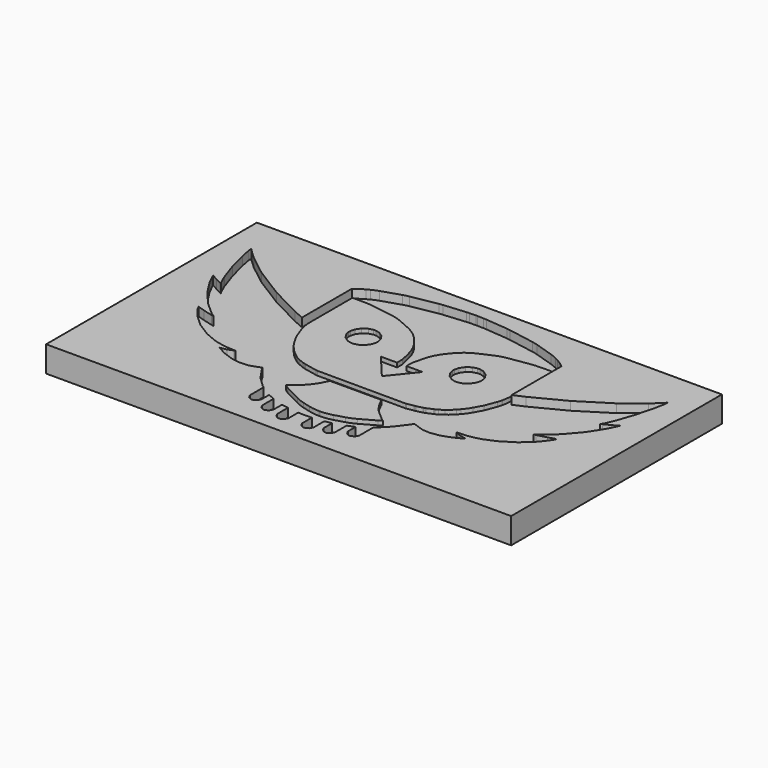
from build123d import *

# Parameters (mm, degrees)
F0_W         = 54.0378913283
F0_H         = 30.6113883853
F1_DEPTH     = 3
F3_DEPTH     = 1
F4_DEPTH     = 0.5
F5_T1_DEPTH  = 1.4279951692
F5_T3_DEPTH  = 1.2750830795
F5_T5_DEPTH  = 1.4154747072
F5_T7_DEPTH  = 1.5538784875
F5_T9_DEPTH  = 1.5346197721
F5_T11_DEPTH = 1.8207083396
F5_T13_DEPTH = 1.842360331
F5_T15_DEPTH = 2.0618682494
F5_T17_DEPTH = 2.9056600537
F5_T19_DEPTH = 2.0631169342
F5_T21_DEPTH = 2.918698365
F5_T23_DEPTH = 2.247874979
F5_T25_DEPTH = 2.5072646643
F5_T27_DEPTH = 3.2701181572
F5_T29_DEPTH = 3.5518654723
F5_T31_DEPTH = 2.1420463635
F5_T33_DEPTH = 3.251600212
F5_T35_DEPTH = 3.5501799152
F5_T37_DEPTH = 2.1451171913
F5_T39_DEPTH = 1.2435255605
F5_T41_DEPTH = 1.2450054051
F5_T43_DEPTH = 2.1117868823
F5_T45_DEPTH = 2.2921133442
F5_T47_DEPTH = 1.9025172431
F5_T49_DEPTH = 1.8626989409
F5_T51_DEPTH = 1.7955373145
F5_T53_DEPTH = 1.8853577819
F5_T55_DEPTH = 1.8365367416
F5_T57_DEPTH = 1.9053253307


# Not quite as in the source:
# - a fillet or chamfer that OpenCascade refuses, or shapes differently, is made with other operations: its cross-section is extruded or revolved along the edge and cut away or added


with BuildPart() as f1:
    # F0 (on Top) → F1 (new body)
    with BuildSketch(Plane.XY):
        Rectangle(F0_W, F0_H)
    extrude(amount=F1_DEPTH)

    # F2 (on face) → F3 (cut)
    with BuildSketch(Plane.XY.offset(3)):
        Polygon((18.8432186, -1.4614652), (18.5729626, -1.5221204), (19.0911226, -1.1666728), (20.5160626, 0.0916432), (21.9755466, 1.7893792), (23.0050086, 3.3946592), (23.5104686, 4.3842432), (23.6539786, 4.7230792), (23.5668566, 4.6707552), (22.9813866, 4.3496992), (22.1975426, 3.9626032), (22.0126306, 3.8757352), (22.2041466, 4.0946832), (22.6712526, 5.1599592), (23.3743246, 7.2338692), (23.9392206, 9.4015052), (24.1762026, 10.6240072), (24.1833146, 10.9671612), (23.9239806, 10.6831892), (22.9346506, 9.7543112), (20.6303626, 7.9450692), (17.1053506, 5.7291732), (13.4495286, 3.8439852), (12.1968006, 3.2940752), (12.1968006, 10.4639872), (12.1968006, 10.5163112), (11.8302786, 10.8884212), (10.3680006, 11.6438172), (7.4962766, 12.5546612), (3.9245286, 13.1899152), (0.9809226, 13.4571232), (-2.54e-05, 13.4807452), (-0.9812274, 13.4611872), (-3.9192708, 13.2008372), (-7.4718418, 12.5655832), (-10.3257604, 11.6466112), (-11.7809518, 10.8871512), (-12.1447814, 10.5163112), (-12.1447814, 10.4901492), (-12.1709688, 10.4901492), (-12.1709688, 3.2940752), (-13.4249668, 3.8439852), (-17.085056, 5.7291732), (-20.618323, 7.9450692), (-22.9320598, 9.7543112), (-23.9256316, 10.6831892), (-24.1833146, 10.9671612), (-24.1778028, 10.6171492), (-23.942167, 9.3905832), (-23.3771694, 7.2229472), (-22.6729798, 5.1558952), (-22.205823, 4.0946832), (-22.014307, 3.8757352), (-22.2003112, 3.9626032), (-22.9706424, 4.3496992), (-23.5425234, 4.6707552), (-23.627969, 4.7230792), (-23.490174, 4.3870372), (-22.9954582, 3.4058352), (-21.9743274, 1.7990312), (-20.517739, 0.0944372), (-19.0942214, -1.1666728), (-18.5747152, -1.5221204), (-18.8461904, -1.4614652), (-19.9472296, -1.1735308), (-20.7175608, -0.9253728), (-20.823682, -0.8867648), (-20.6266288, -1.2754102), (-19.824573, -2.3379176), (-18.458942, -3.5946842), (-16.8618154, -4.588256), (-15.599537, -5.1298094), (-15.1613108, -5.252466), (-14.9297898, -5.3186076), (-13.8783568, -5.5060088), (-12.985369, -5.5487316), (-12.8324102, -5.5432198), (-12.9192274, -5.602478), (-13.5545068, -5.8463942), (-14.214602, -5.9855608), (-14.313789, -5.9924442), (-14.0616432, -6.1509402), (-13.2610098, -6.5629536), (-12.1516648, -6.9653404), (-11.0327186, -7.1376032), (-10.208641, -7.0921372), (-9.948164, -7.0245986), (-9.876536, -7.003923), (-8.917432, -6.6731896), (-8.8113108, -6.6277236), (-8.6404196, -6.9446902), (-7.707503, -8.3048094), (-6.5885314, -9.385173), (-6.3239396, -9.5643192), (-6.3239396, -11.4439954), (-6.3239396, -11.563858), (-6.1323982, -11.9262652), (-5.7809892, -12.1316242), (-5.6624982, -12.1316242), (-5.5453788, -12.1316242), (-5.1939698, -11.9262652), (-5.0010314, -11.563858), (-5.0010314, -11.4439954), (-5.0010314, -10.438003), (-4.9348898, -10.4710738), (-4.273423, -10.7342686), (-4.2072814, -10.7549442), (-4.2072814, -12.3162822), (-4.2072814, -12.4361702), (-4.0157146, -12.7985774), (-3.664331, -13.003911), (-3.5458146, -13.003911), (-3.4286952, -13.003911), (-3.0772862, -12.7985774), (-2.8843732, -12.4361702), (-2.8843732, -12.3162822), (-2.8843732, -11.205591), (-2.8182062, -11.2179608), (-2.1567648, -11.3309654), (-2.0906232, -11.3378742), (-2.0906232, -12.793091), (-2.0906232, -12.9129536), (-1.8990564, -13.2754116), (-1.5476474, -13.4807198), (-1.4291564, -13.4807198), (-1.312037, -13.4807198), (-0.9606534, -13.2754116), (-0.7676134, -12.9129536), (-0.7676134, -12.793091), (-0.7676134, -11.4963448), (-0.7015734, -11.5018566), (-0.2453894, -11.518392), (0.0784606, -11.5225322), (0.2466086, -11.5225322), (0.7535926, -11.5018566), (0.8198866, -11.4963448), (0.8198866, -12.793091), (0.8198866, -12.9129536), (1.0114026, -13.2754116), (1.3626846, -13.4807198), (1.4813026, -13.4807198), (1.5983966, -13.4807198), (1.9496786, -13.2754116), (2.1427186, -12.9129536), (2.1427186, -12.793091), (2.1427186, -11.3378742), (2.2087586, -11.3309654), (2.8704286, -11.2179608), (2.9364686, -11.205591), (2.9364686, -12.3162822), (2.9364686, -12.4361702), (3.1279846, -12.7985774), (3.4795206, -13.003911), (3.5978846, -13.003911), (3.7149786, -13.003911), (4.0665146, -12.7985774), (4.2593006, -12.4361702), (4.2593006, -12.3162822), (4.2593006, -10.7549442), (4.3255946, -10.7287822), (4.9870106, -10.4641904), (5.0530506, -10.438003), (5.0530506, -11.4439954), (5.0530506, -11.563858), (5.2445666, -11.9262652), (5.5961026, -12.1316242), (5.7147206, -12.1316242), (5.8318146, -12.1316242), (6.1830966, -11.9262652), (6.3761366, -11.563858), (6.3761366, -11.4439954), (6.3761366, -9.5643192), (6.5745106, -9.385173), (7.6354686, -8.3048094), (8.6580726, -6.9446902), (8.8371426, -6.6277236), (8.9417906, -6.6731896), (9.8749866, -7.003923), (9.9478846, -7.0245986), (10.2069646, -7.0921372), (11.0309406, -7.1376032), (12.1500646, -6.9653404), (13.2595366, -6.5629536), (14.0598906, -6.1509402), (14.3136366, -5.9924442), (14.2143226, -5.9855608), (13.5516366, -5.8463942), (12.9176526, -5.602478), (12.8323086, -5.5432198), (12.9836926, -5.5487316), (13.8754866, -5.5060088), (14.9280626, -5.3186076), (15.1594566, -5.252466), (15.5953206, -5.1298094), (16.8587166, -4.5923708), (18.4573926, -3.6043108), (19.8213726, -2.3489158), (20.6250286, -1.2782042), (20.8218786, -0.8867648), (20.7157066, -0.9253728), (19.9455786, -1.1735308), align=None)
        Polygon((-5.1278282, -7.5675744), (-5.6363108, -7.2106536), (-5.4778402, -7.1169276), (-4.7598838, -6.5643252), (-4.135628, -5.9194192), (-4.0226488, -5.7816242), (-3.930269, -5.6686196), (-3.5003486, -5.0622708), (-3.0965902, -4.2864532), (-3.0166564, -4.088003), (2.9887926, -4.088003), (3.0672786, -4.2864532), (3.4711386, -5.0622708), (3.9011606, -5.6686196), (3.9948866, -5.7816242), (4.1132506, -5.9263026), (5.4556406, -7.096252), (5.6085486, -7.1830692), (5.2638706, -7.4338942), (3.1142686, -8.6314026), (0.7370826, -9.3273372), (-0.0538734, -9.3273372), (-0.7193534, -9.3273372), (-2.7162252, -8.8036654), align=None, mode=Mode.SUBTRACT)
        Polygon((5.1978306, -3.2542988), (5.1053746, -3.268091), (-5.1333146, -3.2419036), (-5.2986686, -3.221228), (-6.7938396, -2.916682), (-6.933057, -2.871216), (-6.959219, -2.871216), (-6.9798946, -2.871216), (-7.0391274, -2.8450286), (-7.0653402, -2.8450286), (-7.1452486, -2.8174442), (-7.799832, -2.5528524), (-7.8590902, -2.5266904), (-7.8590902, -2.519807), (-7.8797658, -2.500503), (-7.8852776, -2.500503), (-8.2063336, -2.3351236), (-9.0841576, -1.6819626), (-10.0722176, -0.5657088), (-10.8659676, 0.8742172), (-11.360658, 2.2054312), (-11.4833146, 2.6588212), (-11.4971068, 2.7126692), (-11.6156232, 3.0957012), (-11.6156232, 3.2404812), (-11.6156232, 9.9349052), (-10.504932, 9.9349052), (-9.3749114, 9.8922332), (-5.9959748, 9.3588332), (-2.8857448, 7.9780892), (-1.0846308, 5.7235852), (-0.5031994, 3.3258252), (-0.5031994, 2.5264872), (-2.381377, 2.5264872), (0.0784606, -0.4100068), (2.4597106, 2.5264872), (0.5813806, 2.5264872), (0.5854446, 3.3270952), (1.1726926, 5.7235852), (2.9722826, 7.9780892), (6.0769246, 9.3588332), (9.4518226, 9.8922332), (10.5833926, 9.9349052), (11.7200426, 9.9349052), (11.7200426, 3.2404812), (11.7200426, 3.1094172), (11.5739926, 2.7126692), (11.5615466, 2.6588212), (11.4335306, 2.2013672), (10.9275626, 0.8605012), (10.1228906, -0.5850128), (9.1239086, -1.6971264), (8.2336386, -2.3406608), (7.9113126, -2.500503), (7.9042006, -2.5060148), (7.8574646, -2.5266904), (7.7967586, -2.5528524), (7.1630286, -2.8174442), (7.0898766, -2.8450286), (7.0761606, -2.8505404), (6.9699886, -2.8904946), (6.9575426, -2.897378), (6.9313806, -2.897378), (6.8584826, -2.916682), (6.1775086, -3.0958282), (6.1114686, -3.1096204), (6.1046106, -3.1096204), (6.0853066, -3.1096204), (6.0121546, -3.1219902), align=None, mode=Mode.SUBTRACT)
        Polygon((-4.4195238, 4.4297092), (-4.4195238, 4.5909992), (-4.4195238, 4.7507652), (-4.5504354, 5.2262532), (-4.903216, 5.7484772), (-5.4240938, 6.1012832), (-5.9009026, 6.2308232), (-6.0593732, 6.2308232), (-6.2192154, 6.2308232), (-6.6960242, 6.1012832), (-7.216902, 5.7484772), (-7.5696826, 5.2262532), (-7.6992226, 4.7507652), (-7.6992226, 4.5909992), (-7.6992226, 4.4325032), (-7.5696826, 3.9554912), (-7.216902, 3.4332672), (-6.6960242, 3.0804612), (-6.2192154, 2.9496512), (-6.0593732, 2.9496512), (-5.9009026, 2.9496512), (-5.4240938, 3.0763972), (-4.903216, 3.4236152), (-4.5504354, 3.9445692), align=None)
        Polygon((5.8991246, 2.9234892), (6.0591446, 2.9234892), (6.2176406, 2.9234892), (6.6943986, 3.0542992), (7.2153526, 3.4071052), (7.5681586, 3.9280592), (7.6989686, 4.4048172), (7.6989686, 4.5633132), (7.6989686, 4.7230792), (7.5681586, 5.1998372), (7.2153526, 5.7223152), (6.6943986, 6.0751212), (6.2176406, 6.2046612), (6.0591446, 6.2046612), (5.8991246, 6.2046612), (5.4223666, 6.0751212), (4.9001426, 5.7223152), (4.5473366, 5.1998372), (4.4177966, 4.7230792), (4.4177966, 4.5633132), (4.4177966, 4.4048172), (4.5473366, 3.9280592), (4.9001426, 3.4071052), (5.4223666, 3.0542992), align=None)
    extrude(amount=-F3_DEPTH, mode=Mode.SUBTRACT)

    # F4 (cut): faces of the model
    f4_faces = [f1.faces().sort_by_distance(p)[0] for p in [
        (4.6335561224, 8.4234783668, 3),
        (-0.0086091265, -6.6521338784, 3),
    ]]
    extrude(f4_faces, amount=-F4_DEPTH, mode=Mode.SUBTRACT)

    # F5: fillet of radius 5 on 29 edges, made by hand

    # F5_s2 → F5_t1 (join)
    with BuildSketch(Plane.XY.offset(1.5720048308)):
        with BuildLine():
            ThreePointArc((-0.8100633317, 13.4645989611), (-0.9810687986, 13.4582614763), (-1.1517572483, 13.4460759712))
            Line((-1.1517572483, 13.4460759712), (-0.9812274, 13.4611872))
            Line((-0.9812274, 13.4611872), (-0.8100633317, 13.4645989611))
        make_face()
    extrude(amount=F5_T1_DEPTH)

    # F5_s4 → F5_t3 (join)
    with BuildSketch(Plane.XY.offset(1.7249169205)):
        with BuildLine():
            ThreePointArc((0.1099759424, 13.4780962811), (-2.79096e-05, 13.4795346179), (-0.1100367795, 13.4785523767))
            Line((-0.1100367795, 13.4785523767), (-2.54e-05, 13.4807452))
            Line((-2.54e-05, 13.4807452), (0.1099759424, 13.4780962811))
        make_face()
    extrude(amount=F5_T3_DEPTH)

    # F5_s6 → F5_t5 (join)
    with BuildSketch(Plane.XY.offset(1.5845252928)):
        with BuildLine():
            ThreePointArc((1.1464319639, 13.4420989657), (0.9807644678, 13.4543665866), (0.8147808816, 13.4611240234))
            Line((0.8147808816, 13.4611240234), (0.9809226, 13.4571232))
            Line((0.9809226, 13.4571232), (1.1464319639, 13.4420989657))
        make_face()
    extrude(amount=F5_T5_DEPTH)

    # F5_s8 → F5_t7 (join)
    with BuildSketch(Plane.XY.offset(1.4461215125)):
        with BuildLine():
            ThreePointArc((-3.6985841633, 13.2203929921), (-3.918621846, 13.1959742145), (-4.137362893, 13.161839))
            Line((-4.137362893, 13.161839), (-3.9192708, 13.2008372))
            Line((-3.9192708, 13.2008372), (-3.6985841633, 13.2203929921))
        make_face()
    extrude(amount=F5_T7_DEPTH)

    # F5_s10 → F5_t9 (join)
    with BuildSketch(Plane.XY.offset(1.4653802279)):
        with BuildLine():
            ThreePointArc((3.7115563615, 13.2092479116), (3.9239212188, 13.1853847298), (4.1350724232, 13.1524688836))
            Line((4.1350724232, 13.1524688836), (3.9245286, 13.1899152))
            Line((3.9245286, 13.1899152), (3.7115563615, 13.2092479116))
        make_face()
    extrude(amount=F5_T9_DEPTH)

    # F5_s12 → F5_t11 (join)
    with BuildSketch(Plane.XY.offset(1.1792916604)):
        with BuildLine():
            ThreePointArc((7.8091969967, 12.4554101349), (7.4937011449, 12.544208402), (7.1730654496, 12.6121459879))
            Line((7.1730654496, 12.6121459879), (7.4962766, 12.5546612))
            Line((7.4962766, 12.5546612), (7.8091969967, 12.4554101349))
        make_face()
    extrude(amount=F5_T11_DEPTH)

    # F5_s14 → F5_t13 (join)
    with BuildSketch(Plane.XY.offset(1.157639669)):
        with BuildLine():
            ThreePointArc((-7.1401587111, 12.6248932065), (-7.4690995918, 12.5545794677), (-7.7925684671, 12.4623080657))
            Line((-7.7925684671, 12.4623080657), (-7.4718418, 12.5655832))
            Line((-7.4718418, 12.5655832), (-7.1401587111, 12.6248932065))
        make_face()
    extrude(amount=F5_T13_DEPTH)

    # F5_s16 → F5_t15 (join)
    with BuildSketch(Plane.XY.offset(0.9381317506)):
        with BuildLine():
            ThreePointArc((-9.9214566217, 11.7767984631), (-10.3188095179, 11.6299981099), (-10.7023105403, 11.4500908182))
            Line((-10.7023105403, 11.4500908182), (-10.3257604, 11.6466112))
            Line((-10.3257604, 11.6466112), (-9.9214566217, 11.7767984631))
        make_face()
    extrude(amount=F5_T15_DEPTH)

    # F5_s18 → F5_t17 (join)
    with BuildSketch(Plane.XY.offset(0.0943399463)):
        with BuildLine():
            ThreePointArc((-11.1051838212, 11.2398324687), (-11.6479853297, 10.9111234834), (-12.1447814, 10.5163112))
            Line((-12.1447814, 10.5163112), (-11.7809518, 10.8871512))
            Line((-11.7809518, 10.8871512), (-11.1051838212, 11.2398324687))
        make_face()
    extrude(amount=F5_T17_DEPTH)

    # F5_s20 → F5_t19 (join)
    with BuildSketch(Plane.XY.offset(0.9368830658)):
        with BuildLine():
            ThreePointArc((10.7458128931, 11.4486437139), (10.3611047307, 11.627135416), (9.9626544414, 11.7723835652))
            Line((9.9626544414, 11.7723835652), (10.3680006, 11.6438172))
            Line((10.3680006, 11.6438172), (10.7458128931, 11.4486437139))
        make_face()
    extrude(amount=F5_T19_DEPTH)

    # F5_s22 → F5_t21 (join)
    with BuildSketch(Plane.XY.offset(0.081301635)):
        with BuildLine():
            ThreePointArc((12.1968006, 10.5163112), (11.695774938, 10.9120249966), (11.1484083318, 11.2406675397))
            Line((11.1484083318, 11.2406675397), (11.8302786, 10.8884212))
            Line((11.8302786, 10.8884212), (12.1968006, 10.5163112))
        make_face()
    extrude(amount=F5_T21_DEPTH)

    # F5_s24 → F5_t23 (cut)
    with BuildSketch(Plane.XY.offset(2)):
        with BuildLine():
            ThreePointArc((-11.6156232, 3.7948511916), (-11.5859057875, 3.2505250026), (-11.4971068, 2.7126692))
            Line((-11.4971068, 2.7126692), (-11.6156232, 3.0957012))
            Line((-11.6156232, 3.0957012), (-11.6156232, 3.7948511916))
        make_face()
    extrude(amount=F5_T23_DEPTH, mode=Mode.SUBTRACT)

    # F5_s26 → F5_t25 (cut)
    with BuildSketch(Plane.XY.offset(2)):
        with BuildLine():
            ThreePointArc((11.7200426, 3.9123230657), (11.6833958012, 3.3080673251), (11.5739926, 2.7126692))
            Line((11.5739926, 2.7126692), (11.7200426, 3.1094172))
            Line((11.7200426, 3.1094172), (11.7200426, 3.9123230657))
        make_face()
    extrude(amount=F5_T25_DEPTH, mode=Mode.SUBTRACT)

    # F5_s28 → F5_t27 (cut)
    with BuildSketch(Plane.XY.offset(2)):
        with BuildLine():
            ThreePointArc((-0.8235085604, 4.6467454195), (-1.1935422662, 5.670169038), (-1.7762394596, 6.5892908074))
            Line((-1.7762394596, 6.5892908074), (-1.0846308, 5.7235852))
            Line((-1.0846308, 5.7235852), (-0.8235085604, 4.6467454195))
        make_face()
    extrude(amount=F5_T27_DEPTH, mode=Mode.SUBTRACT)

    # F5_s30 → F5_t29 (cut)
    with BuildSketch(Plane.XY.offset(2)):
        with BuildLine():
            ThreePointArc((-2.1237929739, 7.0243331136), (-2.9754726001, 7.8618209534), (-4.0014870822, 8.4734077011))
            Line((-4.0014870822, 8.4734077011), (-2.8857448, 7.9780892))
            Line((-2.8857448, 7.9780892), (-2.1237929739, 7.0243331136))
        make_face()
    extrude(amount=F5_T29_DEPTH, mode=Mode.SUBTRACT)

    # F5_s32 → F5_t31 (cut)
    with BuildSketch(Plane.XY.offset(2)):
        with BuildLine():
            ThreePointArc((-5.3956532676, 9.0923286798), (-6.0081423578, 9.3176359388), (-6.644759274, 9.4612505222))
            Line((-6.644759274, 9.4612505222), (-5.9959748, 9.3588332))
            Line((-5.9959748, 9.3588332), (-5.3956532676, 9.0923286798))
        make_face()
    extrude(amount=F5_T31_DEPTH, mode=Mode.SUBTRACT)

    # F5_s34 → F5_t33 (cut)
    with BuildSketch(Plane.XY.offset(2)):
        with BuildLine():
            ThreePointArc((1.859322928, 6.5837871466), (1.2801170199, 5.6707650681), (0.9107364041, 4.654572783))
            Line((0.9107364041, 4.654572783), (1.1726926, 5.7235852))
            Line((1.1726926, 5.7235852), (1.859322928, 6.5837871466))
        make_face()
    extrude(amount=F5_T33_DEPTH, mode=Mode.SUBTRACT)

    # F5_s36 → F5_t35 (cut)
    with BuildSketch(Plane.XY.offset(2)):
        with BuildLine():
            ThreePointArc((4.0870780672, 8.4738781356), (3.0619754321, 7.8619959383), (2.2111451257, 7.024545626))
            Line((2.2111451257, 7.024545626), (2.9722826, 7.9780892))
            Line((2.9722826, 7.9780892), (4.0870780672, 8.4738781356))
        make_face()
    extrude(amount=F5_T35_DEPTH, mode=Mode.SUBTRACT)

    # F5_s38 → F5_t37 (cut)
    with BuildSketch(Plane.XY.offset(2)):
        with BuildLine():
            ThreePointArc((5.4756586948, 9.0914290062), (6.0891551212, 9.3174875702), (6.7269034579, 9.4615618522))
            Line((6.7269034579, 9.4615618522), (6.0769246, 9.3588332))
            Line((6.0769246, 9.3588332), (5.4756586948, 9.0914290062))
        make_face()
    extrude(amount=F5_T37_DEPTH, mode=Mode.SUBTRACT)

    # F5_s40 → F5_t39 (cut)
    with BuildSketch(Plane.XY.offset(2)):
        with BuildLine():
            ThreePointArc((-9.0811390374, 9.845858202), (-9.3757686657, 9.8834374031), (-9.6721098003, 9.9034560486))
            Line((-9.6721098003, 9.9034560486), (-9.3749114, 9.8922332))
            Line((-9.3749114, 9.8922332), (-9.0811390374, 9.845858202))
        make_face()
    extrude(amount=F5_T39_DEPTH, mode=Mode.SUBTRACT)

    # F5_s42 → F5_t41 (cut)
    with BuildSketch(Plane.XY.offset(2)):
        with BuildLine():
            ThreePointArc((9.1574741093, 9.8457116503), (9.4526838643, 9.8834024437), (9.7496130967, 9.90346301))
            Line((9.7496130967, 9.90346301), (9.4518226, 9.8922332))
            Line((9.4518226, 9.8922332), (9.1574741093, 9.8457116503))
        make_face()
    extrude(amount=F5_T41_DEPTH, mode=Mode.SUBTRACT)

    # F5_s44 → F5_t43 (cut)
    with BuildSketch(Plane.XY.offset(2)):
        with BuildLine():
            ThreePointArc((-1.342980343, -9.1637934794), (-0.7140597146, -9.2862827228), (-0.0746386471, -9.3273372))
            Line((-0.0746386471, -9.3273372), (-0.7193534, -9.3273372))
            Line((-0.7193534, -9.3273372), (-1.342980343, -9.1637934794))
        make_face()
    extrude(amount=F5_T43_DEPTH, mode=Mode.SUBTRACT)

    # F5_s46 → F5_t45 (cut)
    with BuildSketch(Plane.XY.offset(2)):
        with BuildLine():
            ThreePointArc((0.0202372623, -9.3273372), (0.7298269962, -9.2767293253), (1.4250523987, -9.1259301638))
            Line((1.4250523987, -9.1259301638), (0.7370826, -9.3273372))
            Line((0.7370826, -9.3273372), (0.0202372623, -9.3273372))
        make_face()
    extrude(amount=F5_T45_DEPTH, mode=Mode.SUBTRACT)

    # F5_s48 → F5_t47 (cut)
    with BuildSketch(Plane.XY.offset(2)):
        with BuildLine():
            ThreePointArc((2.57585985, -8.7890247962), (3.1021511242, -8.6024626249), (3.6043585701, -8.3583814287))
            Line((3.6043585701, -8.3583814287), (3.1142686, -8.6314026))
            Line((3.1142686, -8.6314026), (2.57585985, -8.7890247962))
        make_face()
    extrude(amount=F5_T47_DEPTH, mode=Mode.SUBTRACT)

    # F5_s50 → F5_t49 (cut)
    with BuildSketch(Plane.XY.offset(2)):
        with BuildLine():
            ThreePointArc((-3.2012978446, -8.5550366123), (-2.7056495399, -8.7759940717), (-2.188974492, -8.9419348309))
            Line((-2.188974492, -8.9419348309), (-2.7162252, -8.8036654))
            Line((-2.7162252, -8.8036654), (-3.2012978446, -8.5550366123))
        make_face()
    extrude(amount=F5_T49_DEPTH, mode=Mode.SUBTRACT)

    # F5_s52 → F5_t51 (cut)
    with BuildSketch(Plane.XY.offset(2)):
        with BuildLine():
            ThreePointArc((-9.4276311884, -1.2939257417), (-9.0660395611, -1.6622379339), (-8.6684049235, -1.9913109818))
            Line((-8.6684049235, -1.9913109818), (-9.0841576, -1.6819626))
            Line((-9.0841576, -1.6819626), (-9.4276311884, -1.2939257417))
        make_face()
    extrude(amount=F5_T51_DEPTH, mode=Mode.SUBTRACT)

    # F5_s54 → F5_t53 (cut)
    with BuildSketch(Plane.XY.offset(2)):
        with BuildLine():
            ThreePointArc((-10.3397327852, -0.0804148529), (-10.0471985593, -0.5480665606), (-9.7049307583, -0.9806485129))
            Line((-9.7049307583, -0.9806485129), (-10.0722176, -0.5657088))
            Line((-10.0722176, -0.5657088), (-10.3397327852, -0.0804148529))
        make_face()
    extrude(amount=F5_T53_DEPTH, mode=Mode.SUBTRACT)

    # F5_s56 → F5_t55 (cut)
    with BuildSketch(Plane.XY.offset(2)):
        with BuildLine():
            ThreePointArc((9.4811674098, -1.2994091428), (9.1048514826, -1.6759348967), (8.6906373407, -2.0103178586))
            Line((8.6906373407, -2.0103178586), (9.1239086, -1.6971264))
            Line((9.1239086, -1.6971264), (9.4811674098, -1.2994091428))
        make_face()
    extrude(amount=F5_T55_DEPTH, mode=Mode.SUBTRACT)

    # F5_s58 → F5_t57 (cut)
    with BuildSketch(Plane.XY.offset(2)):
        with BuildLine():
            ThreePointArc((10.3963027069, -0.0938548769), (10.0972518382, -0.5667127565), (9.7472444697, -1.0031996846))
            Line((9.7472444697, -1.0031996846), (10.1228906, -0.5850128))
            Line((10.1228906, -0.5850128), (10.3963027069, -0.0938548769))
        make_face()
    extrude(amount=F5_T57_DEPTH, mode=Mode.SUBTRACT)


solid = f1.part
